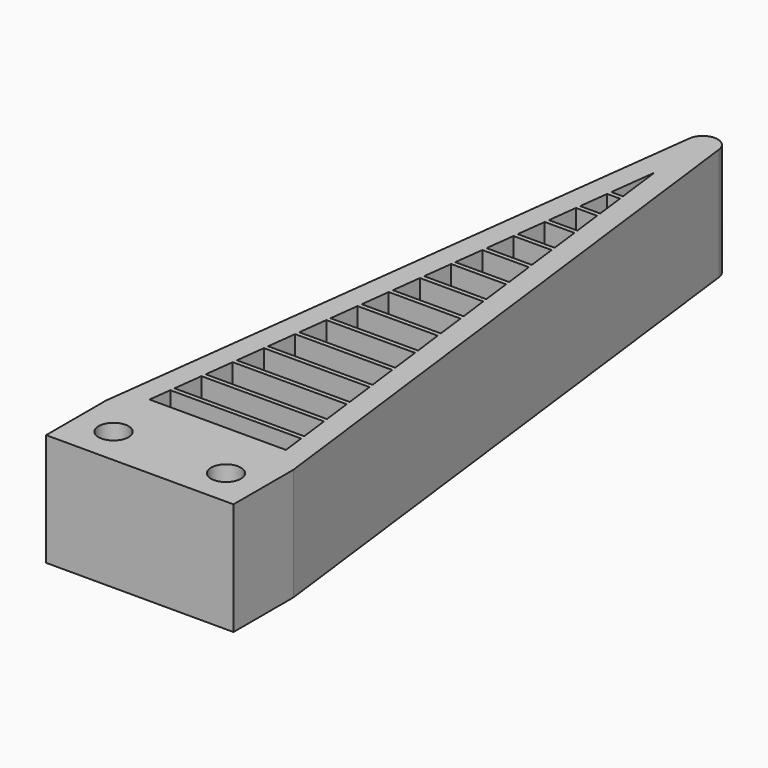
from build123d import *

# Parameters (mm, degrees)
F0_W     = 25
F0_H     = 10
F0_R     = 2
F1_DEPTH = 7.5
F2_R     = 2


# Not quite as in the source:
# - a feature names something its author has since deleted; it is built from what else it names


with BuildPart() as f1:
    # F0 (on Top) → F1 (new body, symmetric)
    with BuildSketch(Plane.XY):
        Polygon((17.8516533444, 33), (20.875, 33), (20.8, 33.6), (17.7766533444, 33.6), align=None)
        Polygon((17.7766533444, 33.6), (20.8, 33.6), (20.3125, 37.5), (17.2891533444, 37.5), align=None)
        Polygon((17.2891533444, 37.5), (20.3125, 37.5), (20.2375, 38.1), (17.2141533444, 38.1), align=None)
        Polygon((17.2141533444, 38.1), (20.2375, 38.1), (19.75, 42), (16.7266533444, 42), align=None)
        Polygon((16.7266533444, 42), (19.75, 42), (19.675, 42.6), (16.6516533444, 42.6), align=None)
        Polygon((16.6516533444, 42.6), (19.675, 42.6), (19.1875, 46.5), (16.1641533444, 46.5), align=None)
        Polygon((16.1641533444, 46.5), (19.1875, 46.5), (19.1125, 47.1), (16.0891533444, 47.1), align=None)
        Polygon((16.0891533444, 47.1), (19.1125, 47.1), (18.625, 51), (15.6016533444, 51), align=None)
        Polygon((15.6016533444, 51), (18.625, 51), (18.55, 51.6), (15.5266533444, 51.6), align=None)
        Polygon((15.5266533444, 51.6), (18.55, 51.6), (18.0625, 55.5), (15.0391533444, 55.5), align=None)
        Polygon((15.0391533444, 55.5), (18.0625, 55.5), (17.9875, 56.1), (14.9641533444, 56.1), align=None)
        Polygon((14.9641533444, 56.1), (17.9875, 56.1), (17.5, 60), (14.4766533444, 60), align=None)
        Polygon((14.4766533444, 60), (17.5, 60), (17.425, 60.6), (14.4016533444, 60.6), align=None)
        Polygon((14.4016533444, 60.6), (17.425, 60.6), (16.9375, 64.5), (13.9141533444, 64.5), align=None)
        Polygon((13.9141533444, 64.5), (16.9375, 64.5), (16.8625, 65.1), (13.8391533444, 65.1), align=None)
        Polygon((13.8391533444, 65.1), (16.8625, 65.1), (16.375, 69), (13.3516533444, 69), align=None)
        Polygon((13.3516533444, 69), (16.375, 69), (16.3, 69.6), (13.2766533444, 69.6), align=None)
        Polygon((12.5, 100), (8.7, 69.6), (11.7233466556, 69.6), (12.5, 75.8132267551), (13.2766533444, 69.6), (16.3, 69.6), align=None)
        with Locations((12.5, -5)):
            Rectangle(F0_W, F0_H)
        with Locations((5, -5)):
            Circle(F0_R, mode=Mode.SUBTRACT)
        with Locations((20, -5)):
            Circle(F0_R, mode=Mode.SUBTRACT)
        Polygon((8.0625, 64.5), (7.575, 60.6), (10.5983466556, 60.6), (11.0858466556, 64.5), align=None)
        Polygon((8.7, 69.6), (8.625, 69), (11.6483466556, 69), (11.7233466556, 69.6), align=None)
        Polygon((8.1375, 65.1), (8.0625, 64.5), (11.0858466556, 64.5), (11.1608466556, 65.1), align=None)
        Polygon((8.625, 69), (8.1375, 65.1), (11.1608466556, 65.1), (11.6483466556, 69), align=None)
        Polygon((6.375, 51), (5.8875, 47.1), (8.9108466556, 47.1), (9.3983466556, 51), align=None)
        Polygon((7.5, 60), (7.0125, 56.1), (10.0358466556, 56.1), (10.5233466556, 60), align=None)
        Polygon((7.0125, 56.1), (6.9375, 55.5), (9.9608466556, 55.5), (10.0358466556, 56.1), align=None)
        Polygon((7.575, 60.6), (7.5, 60), (10.5233466556, 60), (10.5983466556, 60.6), align=None)
        Polygon((6.45, 51.6), (6.375, 51), (9.3983466556, 51), (9.4733466556, 51.6), align=None)
        Polygon((6.9375, 55.5), (6.45, 51.6), (9.4733466556, 51.6), (9.9608466556, 55.5), align=None)
        Polygon((5.25, 42), (4.7625, 38.1), (7.7858466556, 38.1), (8.2733466556, 42), align=None)
        Polygon((4.2, 33.6), (4.125, 33), (7.1483466556, 33), (7.2233466556, 33.6), align=None)
        Polygon((5.325, 42.6), (5.25, 42), (8.2733466556, 42), (8.3483466556, 42.6), align=None)
        Polygon((5.8125, 46.5), (5.325, 42.6), (8.3483466556, 42.6), (8.8358466556, 46.5), align=None)
        Polygon((4.6875, 37.5), (4.2, 33.6), (7.2233466556, 33.6), (7.7108466556, 37.5), align=None)
        Polygon((4.125, 33), (0, 0), (25, 0), (20.875, 33), (17.8516533444, 33), (18.3391533444, 29.1), (18.4141533444, 28.5), (18.9016533444, 24.6), (18.9766533444, 24), (19.4641533444, 20.1), (19.5391533444, 19.5), (20.0266533444, 15.6), (20.1016533444, 15), (20.5891533444, 11.1), (20.6641533444, 10.5), (21.1516533444, 6.6), (21.2266533444, 6), (21.6016533444, 3), (3.3983466556, 3), (3.7733466556, 6), (3.8483466556, 6.6), (4.3358466556, 10.5), (4.4108466556, 11.1), (4.8983466556, 15), (4.9733466556, 15.6), (5.4608466556, 19.5), (5.5358466556, 20.1), (6.0233466556, 24), (6.0983466556, 24.6), (6.5858466556, 28.5), (6.6608466556, 29.1), (7.1483466556, 33), align=None)
        Polygon((5.8875, 47.1), (5.8125, 46.5), (8.8358466556, 46.5), (8.9108466556, 47.1), align=None)
        Polygon((4.7625, 38.1), (4.6875, 37.5), (7.7108466556, 37.5), (7.7858466556, 38.1), align=None)
        Polygon((21.1516533444, 6.6), (3.8483466556, 6.6), (3.7733466556, 6), (21.2266533444, 6), align=None)
        Polygon((20.5891533444, 11.1), (4.4108466556, 11.1), (4.3358466556, 10.5), (20.6641533444, 10.5), align=None)
        Polygon((20.0266533444, 15.6), (4.9733466556, 15.6), (4.8983466556, 15), (20.1016533444, 15), align=None)
        Polygon((19.4641533444, 20.1), (5.5358466556, 20.1), (5.4608466556, 19.5), (19.5391533444, 19.5), align=None)
        Polygon((18.9016533444, 24.6), (6.0983466556, 24.6), (6.0233466556, 24), (18.9766533444, 24), align=None)
        Polygon((18.3391533444, 29.1), (6.6608466556, 29.1), (6.5858466556, 28.5), (18.4141533444, 28.5), align=None)
        Polygon((7.2233466556, 33.6), (7.1483466556, 33), (17.8516533444, 33), (17.7766533444, 33.6), align=None)
        Polygon((7.7858466556, 38.1), (7.7108466556, 37.5), (17.2891533444, 37.5), (17.2141533444, 38.1), align=None)
        Polygon((8.3483466556, 42.6), (8.2733466556, 42), (16.7266533444, 42), (16.6516533444, 42.6), align=None)
        Polygon((8.9108466556, 47.1), (8.8358466556, 46.5), (16.1641533444, 46.5), (16.0891533444, 47.1), align=None)
        Polygon((9.4733466556, 51.6), (9.3983466556, 51), (15.6016533444, 51), (15.5266533444, 51.6), align=None)
        Polygon((10.0358466556, 56.1), (9.9608466556, 55.5), (15.0391533444, 55.5), (14.9641533444, 56.1), align=None)
        Polygon((10.5983466556, 60.6), (10.5233466556, 60), (14.4766533444, 60), (14.4016533444, 60.6), align=None)
        Polygon((11.1608466556, 65.1), (11.0858466556, 64.5), (13.9141533444, 64.5), (13.8391533444, 65.1), align=None)
        Polygon((11.7233466556, 69.6), (11.6483466556, 69), (13.3516533444, 69), (13.2766533444, 69.6), align=None)
    extrude(amount=F1_DEPTH, both=True)

    # F2
    f2_edges = [f1.edges().sort_by_distance(p)[0] for p in [
        (12.5, 100, 0),
    ]]
    fillet(f2_edges, radius=F2_R)


solid = f1.part
